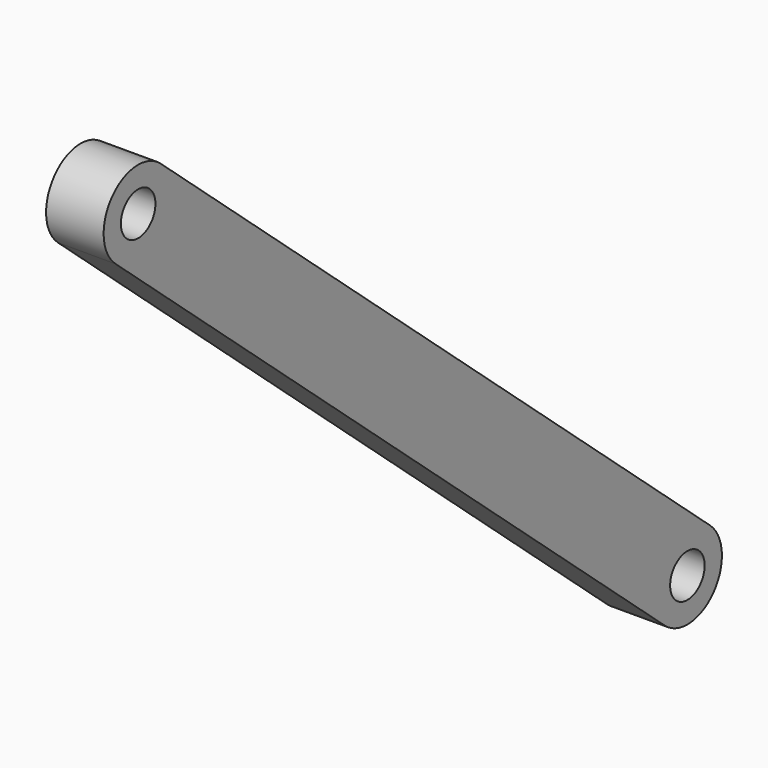
from build123d import *

# Parameters (mm, degrees)
F0_R     = 4.7625
F1_DEPTH = 12.7


# Not quite as in the source:
# - a feature names something its author has since deleted; it is built from what else it names


with BuildPart() as f1:
    # F0 (on Right) → F1 (new body)
    with BuildSketch(Plane.YZ):
        with BuildLine():
            ThreePointArc((135.0932664818, 138.7993858615), (134.1614165409, 152.23749978), (147.5995304594, 153.1693497209))
            Line((147.5995304594, 153.1693497209), (-3.9226998699, 285.0400370456))
            ThreePointArc((-3.9226998699, 285.0400370456), (-1.5073052482, 281.8024937035), (-0.6508318587, 277.8550551158))
            ThreePointArc((-0.6508318587, 277.8550551158), (-6.2283932711, 269.1865285054), (-16.4289638475, 270.6700731861))
            Line((-16.4289638475, 270.6700731861), (135.0932664818, 138.7993858615))
        make_face()
        with BuildLine():
            ThreePointArc((-0.6508318587, 277.8550551158), (-1.5073052482, 281.8024937035), (-3.9226998699, 285.0400370456))
            ThreePointArc((-3.9226998699, 285.0400370456), (-17.3608137885, 284.1081871047), (-16.4289638475, 270.6700731861))
            ThreePointArc((-16.4289638475, 270.6700731861), (-6.2283932711, 269.1865285054), (-0.6508318587, 277.8550551158))
        make_face()
        with Locations((-10.1758318587, 277.8550551158)):
            Circle(F0_R, mode=Mode.SUBTRACT)
        with BuildLine():
            ThreePointArc((135.0932664818, 138.7993858615), (145.2938370582, 137.3158411807), (150.8713984706, 145.9843677912))
            ThreePointArc((150.8713984706, 145.9843677912), (150.0149250811, 149.9318063789), (147.5995304594, 153.1693497209))
            ThreePointArc((147.5995304594, 153.1693497209), (134.1614165409, 152.23749978), (135.0932664818, 138.7993858615))
        make_face()
        with Locations((141.3463984706, 145.9843677912)):
            Circle(F0_R, mode=Mode.SUBTRACT)
    extrude(amount=F1_DEPTH)


solid = f1.part
